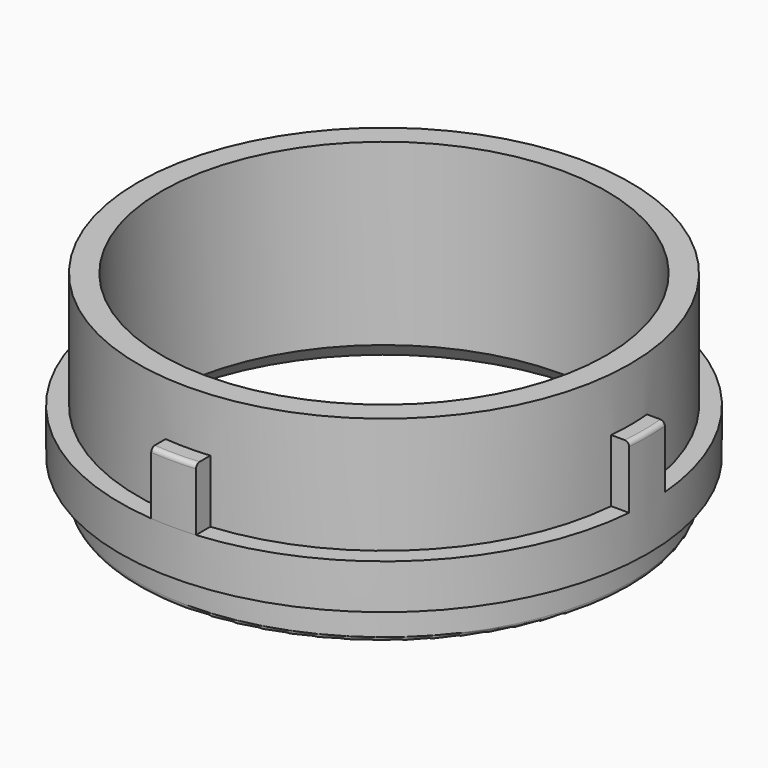
from build123d import *

# Parameters (mm, degrees)
F2_R            = 0.5
F3_SIZE         = 2
F5_DEPTH        = 7
F5_COPIES_COUNT = 4
F6_R            = 0.5


# Not quite as in the source:
# - after a boolean that leaves OpenCascade's solid faulty, fix() repairs it
# - a pattern or mirror of a feature is missing from the dataset's text; its kind, count and spacing are read off the source's solid


with BuildPart() as f1:
    # F0 (on Front) → F1 (revolve)
    with BuildSketch(Plane.XZ):
        Polygon((27.5, 0), (24.85, 0), (24.85, -22), (27.5, -22), (27.5, -18), (29.5, -18), (29.5, -13), (27.5, -13), align=None)
    revolve(axis=Axis((0, 0, -6.1865765601), (0, 0, -1)))

    # F2
    f2_edges = [f1.edges().sort_by_distance(p)[0] for p in [
        (-27.5, 0, -22),
    ]]
    fillet(f2_edges, radius=F2_R)

    # F3
    f3_edges = [f1.edges().sort_by_distance(p)[0] for p in [
        (-24.85, 0, -22),
    ]]
    chamfer(f3_edges, length=F3_SIZE)

    # F4 (on face) → F5 (join)
    with BuildSketch(Plane.XY.offset(-13)):
        with BuildLine():
            Line((-2.5, 29.3938769134), (-2.5, 27.3861278753))
            Line((-2.5, 27.3861278753), (2.5, 27.3861278753))
            Line((2.5, 27.3861278753), (2.5, 29.3938769134))
            ThreePointArc((2.5, 29.3938769134), (0, 29.5), (-2.5, 29.3938769134))
        make_face()
    f5 = extrude(amount=F5_DEPTH)

    # F5_copies: F5 ×4 about axis
    f5_copies_axis = Axis((0, 0, 0), (0, 0, 1))
    for i in range(1, F5_COPIES_COUNT):
        add(f5.rotate(f5_copies_axis, i * 360 / F5_COPIES_COUNT))

    add(f1.part.fix(), mode=Mode.REPLACE)

    # F6
    f6_edges = [f1.edges().sort_by_distance(p)[0] for p in [
        (0, 29.5, -6),
        (-29.5, 0, -6),
        (0, -29.5, -6),
        (29.5, 0, -6),
    ]]
    fillet(f6_edges, radius=F6_R)


solid = f1.part
